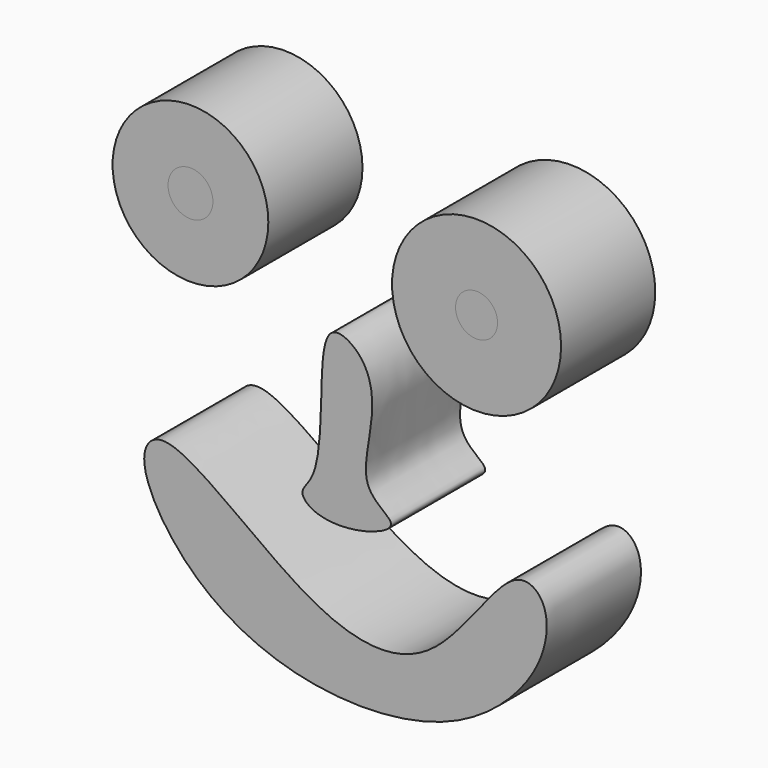
from build123d import *

# Parameters (mm, degrees)
F0_R     = 16.5364036615
F1_DEPTH = 25
F0_R_2   = 17.9507843836
F2_R     = 4.7674221811
F4_DEPTH = 5
F3_R     = 4.4629854582
F5_DEPTH = 5


with BuildPart() as f1:
    # F0 (on Front) → F1 (new body)
    with BuildSketch(Plane.XZ):
        with Locations((-35.8772203326, 37.2763350606)):
            Circle(F0_R)
    extrude(amount=F1_DEPTH)


with BuildPart() as f1b:
    # F0 (on Front) → F1, piece 2 (new body)
    with BuildSketch(Plane.XZ):
        with Locations((24.8842034489, 34.2782363296)):
            Circle(F0_R_2)
    extrude(amount=F1_DEPTH)


with BuildPart() as f1c:
    # F0 (on Front) → F1, piece 3 (new body)
    with BuildSketch(Plane.XZ):
        with BuildLine():
            add(Edge.make_bspline(
                [(-5.6963833049, 21.0866127163), (-7.8834558008, 19.8463029152), (-8.0268802726, 7.5598642764), (-8.6262310867, -7.1486815614), (-13.1603918881, -10.7476265806), (-9.5090955089, -14.4774036327), (-0.5035687728, -14.9780889681), (8.6722579471, -11.2593562384), (4.0459610335, -8.1665176761), (-0.0134878093, -3.8003686921), (3.7817051014, 9.0097780906), (1.5463833673, 18.8922525571), (-4.1892052399, 21.9413478609), (-5.6963833049, 21.0866127163)],
                knots=[0, 0, 0, 0, 0.1173610371, 0.2463343395, 0.3123312978, 0.3735055392, 0.474889194, 0.5635056711, 0.6235237394, 0.6997360761, 0.8154360044, 0.9191229458, 1, 1, 1, 1], degree=3))
        make_face()
    extrude(amount=F1_DEPTH)


with BuildPart() as f1d:
    # F0 (on Front) → F1, piece 4 (new body)
    with BuildSketch(Plane.XZ):
        with BuildLine():
            add(Edge.make_bspline(
                [(-41.2737950683, -10.8930841088), (-34.5995164089, -11.4871246973), (-9.7534140649, -35.3385848681), (16.8616589842, -36.7148668452), (31.2960074258, -9.2465484487), (40.3597191314, -14.1079932129), (39.9817917652, -27.7981943972), (21.2095931844, -47.1750034429), (-13.6794713141, -48.127909166), (-37.8079824477, -34.2926990998), (-48.1586983843, -15.4859918262), (-43.9173012619, -10.6578002594), (-41.2737950683, -10.8930841088)],
                knots=[0, 0, 0, 0, 0.1375136585, 0.2482954713, 0.3616240255, 0.415221879, 0.4906580747, 0.6021038602, 0.7309402294, 0.8491958392, 0.9455344575, 1, 1, 1, 1], degree=3))
        make_face()
    extrude(amount=F1_DEPTH)


with BuildPart() as f4:
    # F2 (on face) → F4 (new body)
    with BuildSketch(Plane.XZ.offset(25)):
        with Locations((-35.8772203326, 37.2763350606)):
            Circle(F2_R)
    extrude(amount=-F4_DEPTH)


with BuildPart() as f4b:
    # F3 (on face) → F4, piece 2 (new body)
    with BuildSketch(Plane.XZ.offset(25)):
        with Locations((24.8842034489, 34.2782363296)):
            Circle(F3_R)
    extrude(amount=-F4_DEPTH)


with BuildPart() as f5:
    # F5 (new): a face of the model
    f5_faces = [f4.part.faces().sort_by_distance(p)[0] for p in [
        (-35.8772203326, -25, 37.2763350606),
    ]]
    extrude(f5_faces, amount=-F5_DEPTH)


solid = Compound([f1.part, f1b.part, f1c.part, f1d.part, f4.part, f4b.part, f5.part])
